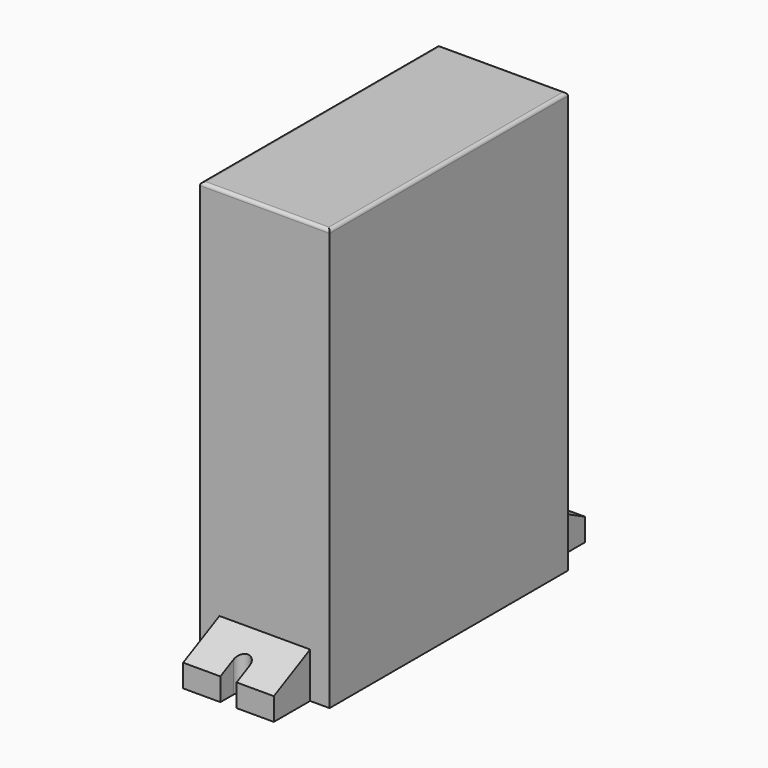
from build123d import *

# Parameters (mm, degrees)
F1_DEPTH      = 20
F1_DEPTH_BACK = 20
F2_DEPTH      = 14
F2_DEPTH_BACK = 14
F4_DEPTH      = 25
F5_ANGLE      = 90
F6_R          = 1


with BuildPart() as f1:
    # F0 (on Right) → F1 (new body, two sides)
    with BuildSketch(Plane.YZ) as f1_sk:
        Polygon((48.225797835, 46), (-67.774202165, 46), (-67.774202165, 0), (62.225797835, 0), (62.225797835, 46), align=None)
        Polygon((62.225797835, 0), (-67.774202165, 0), (-67.774202165, -46), (48.225797835, -46), (62.225797835, -46), align=None)
    extrude(amount=F1_DEPTH)
    extrude(f1_sk.sketch, amount=-F1_DEPTH_BACK)

    # F0 (on Right) → F2 (join, two sides)
    with BuildSketch(Plane.YZ) as f2_sk:
        Polygon((55.225797835, 60), (48.225797835, 46), (62.225797835, 46), (62.225797835, 60), align=None)
        Polygon((62.225797835, -60), (62.225797835, -46), (48.225797835, -46), (55.225797835, -60), align=None)
    extrude(amount=F2_DEPTH)
    extrude(f2_sk.sketch, amount=-F2_DEPTH_BACK)

    # F3 (on face) → F4 (cut)
    with BuildSketch(Plane(origin=(0, 62.225797835, 0), x_dir=(-1, 0, 0), z_dir=(0, 1, 0))):
        with BuildLine():
            Line((2.5, 55), (2.5, 60))
            Line((2.5, 60), (-2.5, 60))
            Line((-2.5, 60), (-2.5, 55))
            ThreePointArc((-2.5, 55), (0, 52.5), (2.5, 55))
        make_face()
        with BuildLine():
            Line((2.5, -60), (2.5, -55))
            ThreePointArc((2.5, -55), (0, -52.5), (-2.5, -55))
            Line((-2.5, -55), (-2.5, -60))
            Line((-2.5, -60), (2.5, -60))
        make_face()
    extrude(amount=-F4_DEPTH, mode=Mode.SUBTRACT)


with BuildPart() as f1_1:
    # F5: moved
    add(f1.part.rotate(Axis((0, -67.774202165, 46), (-1, 0, 0)), F5_ANGLE))

    # F6
    f6_edges = [f1_1.edges().sort_by_distance(p)[0] for p in [
        (0, -159.774202, 46),
        (0, -67.774202, 46),
        (-20, -113.774202, 46),
        (20, -113.774202, 46),
    ]]
    fillet(f6_edges, radius=F6_R)


solid = f1_1.part
